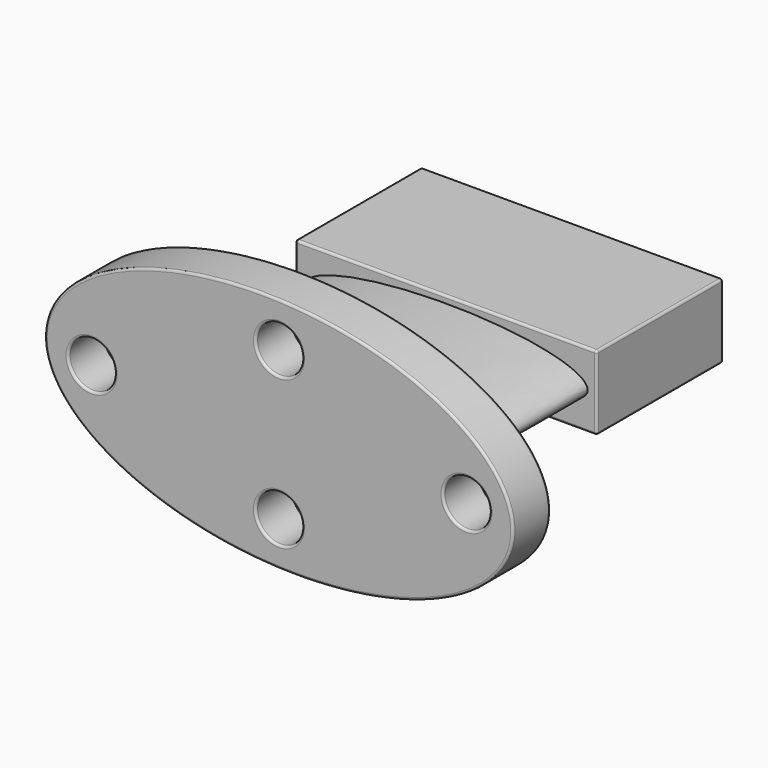
from build123d import *

# Parameters (mm, degrees)
F0_W     = 65
F0_H     = 16
F1_DEPTH = 34
F3_W     = 60.5
F3_H     = 11.5
F4_DEPTH = 32
F5_DEPTH = 35
F7_DEPTH = 10
F8_R     = 5
F9_DEPTH = 10.0010001
F10_R    = 0.5


with BuildPart() as f1:
    # F0 (on Front) → F1 (new body)
    with BuildSketch(Plane.XZ):
        Rectangle(F0_W, F0_H)
    extrude(amount=F1_DEPTH)

    # F3 (on face) → F4 (cut)
    with BuildSketch(Plane(origin=(0, 0, 0), x_dir=(-1, 0, 0), z_dir=(0, 1, 0))):
        Rectangle(F3_W, F3_H)
    extrude(amount=-F4_DEPTH, mode=Mode.SUBTRACT)

    # F2 (on face) → F5 (join)
    with BuildSketch(Plane.XZ.offset(34)):
        with BuildLine():
            add(Edge.make_bspline(
                [(30.5, 0), (30.5, 11.2583302492), (-15.25, 5.6291651246), (-61, 0), (-15.25, -5.6291651246), (30.5, -11.2583302492), (30.5, 0)],
                knots=[0, 0, 0, 2.0943951024, 2.0943951024, 4.1887902048, 4.1887902048, 6.2831853072, 6.2831853072, 6.2831853072], degree=2, weights=[1, 0.5, 1, 0.5, 1, 0.5, 1]))
        make_face()
    extrude(amount=F5_DEPTH)

    # F6 (on face) → F7 (join)
    with BuildSketch(Plane.XZ.offset(69)):
        with BuildLine():
            add(Edge.make_bspline(
                [(50.423003109, -2.7876078398), (52.8610446824, 41.3123462791), (-23.9924807678, 23.4437809793), (-100.846006218, 5.5752156796), (-26.4305223412, -20.6561731395), (47.9849615356, -46.8875619586), (50.423003109, -2.7876078398)],
                knots=[0, 0, 0, 2.0943951024, 2.0943951024, 4.1887902048, 4.1887902048, 6.2831853072, 6.2831853072, 6.2831853072], degree=2, weights=[1, 0.5, 1, 0.5, 1, 0.5, 1]))
        make_face()
        with BuildLine():
            add(Edge.make_bspline(
                [(30.5, 0), (30.5, 11.2583302492), (-15.25, 5.6291651246), (-61, 0), (-15.25, -5.6291651246), (30.5, -11.2583302492), (30.5, 0)],
                knots=[0, 0, 0, 2.0943951024, 2.0943951024, 4.1887902048, 4.1887902048, 6.2831853072, 6.2831853072, 6.2831853072], degree=2, weights=[1, 0.5, 1, 0.5, 1, 0.5, 1]))
        make_face(mode=Mode.SUBTRACT)
        with BuildLine():
            add(Edge.make_bspline(
                [(30.5, 0), (30.5, 11.2583302492), (-15.25, 5.6291651246), (-61, 0), (-15.25, -5.6291651246), (30.5, -11.2583302492), (30.5, 0)],
                knots=[0, 0, 0, 2.0943951024, 2.0943951024, 4.1887902048, 4.1887902048, 6.2831853072, 6.2831853072, 6.2831853072], degree=2, weights=[1, 0.5, 1, 0.5, 1, 0.5, 1]))
        make_face()
    extrude(amount=F7_DEPTH)

    # F8 (on face) → F9 (cut, through all)
    with BuildSketch(Plane(origin=(0, -69, 0), x_dir=(-1, 0, 0), z_dir=(0, 1, 0))):
        with Locations((40.3883401646, 0)):
            Circle(F8_R)
        with Locations((0, 16.0144967895)):
            Circle(F8_R)
        with Locations((-40.3883401646, 0)):
            Circle(F8_R)
        with Locations((0, -16.0144967895)):
            Circle(F8_R)
    extrude(amount=-F9_DEPTH, mode=Mode.SUBTRACT)

    # F10
    f10_edges = [f1.edges().sort_by_distance(p)[0] for p in [
        (0, 0, 8),
        (0, 0, 5.75),
        (30.25, 0, 0),
        (0, 0, -5.75),
        (32.5, 0, 0),
        (0, 0, -8),
        (-32.5, 0, 0),
        (-30.25, 0, 0),
        (-32.5, -17, 8),
        (-32.5, -17, -8),
        (-32.5, -34, 0),
        (0, -34, 8),
        (32.5, -17, 8),
        (32.5, -17, -8),
        (32.5, -34, 0),
        (0, -34, -8),
        (-50.423003, -69, 2.787613),
        (-50.423003, -79, 2.787613),
        (45.38834, -79, 0),
        (5, -79, -16.014497),
        (5, -79, 16.014497),
        (-35.38834, -79, 0),
        (45.38834, -69, 0),
        (5, -69, 16.014497),
        (5, -69, -16.014497),
        (-35.38834, -69, 0),
    ]]
    fillet(f10_edges, radius=F10_R)


solid = f1.part
